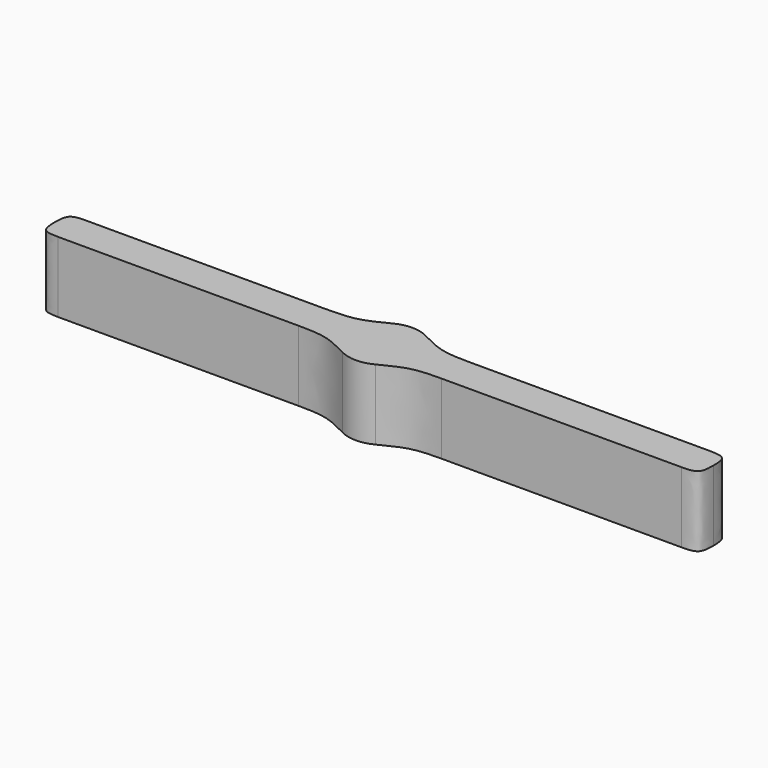
from build123d import *

# Parameters (mm, degrees)
F0_R        = 7.9375
F1_DEPTH    = 38.1
F2_T1_DEPTH = 85.725
F3_T1_DEPTH = 38.1


# Not quite as in the source:
# - a fillet or chamfer that OpenCascade refuses, or shapes differently, is made with other operations: its cross-section is extruded or revolved along the edge and cut away or added
# - a length typed as a fraction of an inch, garbled in the dataset ("3 / 203.2 mm" for 3/8 in), is restored


with BuildPart() as f1:
    # F0 (on Top) → F1 (new body)
    with BuildSketch(Plane.XY):
        with BuildLine():
            Line((16.4977839421, -9.525), (177.8, -9.525))
            Line((177.8, -9.525), (177.8, 9.525))
            Line((177.8, 9.525), (16.4977839421, 9.525))
            ThreePointArc((16.4977839421, 9.525), (0, 19.05), (-16.4977839421, 9.525))
            Line((-16.4977839421, 9.525), (-177.8, 9.525))
            Line((-177.8, 9.525), (-177.8, -9.525))
            Line((-177.8, -9.525), (-16.4977839421, -9.525))
            ThreePointArc((-16.4977839421, -9.525), (0, -19.05), (16.4977839421, -9.525))
        make_face()
        Circle(F0_R, mode=Mode.SUBTRACT)
        Circle(F0_R)
    extrude(amount=F1_DEPTH)

    # F2: fillet of radius 9.525 on 4 edges, made by hand

    # F2_s2 → F2_t1 (cut)
    with BuildSketch(Plane.XY.offset(-23.8125)):
        with BuildLine():
            add(Edge.make_bspline(
                [(-177.8, 0), (-177.8, -9.525), (-168.275, -9.525)],
                knots=[0, 0, 0, 1, 1, 1], degree=2, weights=[1, 1.8571428571, 1]))
            Line((-168.275, -9.525), (-177.8, -9.525))
            Line((-177.8, -9.525), (-177.8, 0))
        make_face()
        with BuildLine():
            add(Edge.make_bspline(
                [(-168.275, 9.525), (-177.8, 9.525), (-177.8, 0)],
                knots=[0, 0, 0, 1, 1, 1], degree=2, weights=[1, 1.8571428571, 1]))
            Line((-177.8, 0), (-177.8, 9.525))
            Line((-177.8, 9.525), (-168.275, 9.525))
        make_face()
        with BuildLine():
            add(Edge.make_bspline(
                [(177.8, 0), (177.8, 9.525), (168.275, 9.525)],
                knots=[0, 0, 0, 1, 1, 1], degree=2, weights=[1, 1.8571428571, 1]))
            Line((168.275, 9.525), (177.8, 9.525))
            Line((177.8, 9.525), (177.8, 0))
        make_face()
        with BuildLine():
            add(Edge.make_bspline(
                [(168.275, -9.525), (177.8, -9.525), (177.8, 0)],
                knots=[0, 0, 0, 1, 1, 1], degree=2, weights=[1, 1.8571428571, 1]))
            Line((177.8, 0), (177.8, -9.525))
            Line((177.8, -9.525), (168.275, -9.525))
        make_face()
    extrude(amount=F2_T1_DEPTH, mode=Mode.SUBTRACT)

    # F3: fillet of radius 64.0333905996 on 4 edges, made by hand

    # F3_s2 → F3_t1 (join)
    with BuildSketch(Plane.XY):
        with BuildLine():
            add(Edge.make_bspline(
                [(8.8566007427, 16.8660346046), (22.8364726227, 9.525), (38.6265836688, 9.525)],
                knots=[0, 0, 0, 1, 1, 1], degree=2, weights=[1, 1.8571428571, 1]))
            Line((38.6265836688, 9.525), (16.4977839421, 9.525))
            ThreePointArc((16.4977839421, 9.525), (13.1978749408, 13.737488746), (8.8566007427, 16.8660346046))
        make_face()
        with BuildLine():
            add(Edge.make_bspline(
                [(-38.6265836688, 9.525), (-22.8364726227, 9.525), (-8.8566007427, 16.8660346046)],
                knots=[0, 0, 0, 1, 1, 1], degree=2, weights=[1, 1.8571428571, 1]))
            ThreePointArc((-8.8566007427, 16.8660346046), (-13.1978749408, 13.737488746), (-16.4977839421, 9.525))
            Line((-16.4977839421, 9.525), (-38.6265836688, 9.525))
        make_face()
        with BuildLine():
            add(Edge.make_bspline(
                [(-8.8566007427, -16.8660346046), (-22.8364726227, -9.525), (-38.6265836688, -9.525)],
                knots=[0, 0, 0, 1, 1, 1], degree=2, weights=[1, 1.8571428571, 1]))
            Line((-38.6265836688, -9.525), (-16.4977839421, -9.525))
            ThreePointArc((-16.4977839421, -9.525), (-13.1978749408, -13.737488746), (-8.8566007427, -16.8660346046))
        make_face()
        with BuildLine():
            add(Edge.make_bspline(
                [(8.8566007427, -16.8660346046), (22.8364726227, -9.525), (38.6265836688, -9.525)],
                knots=[0, 0, 0, 1, 1, 1], degree=2, weights=[1, 1.8571428571, 1]))
            Line((38.6265836688, -9.525), (16.4977839421, -9.525))
            ThreePointArc((16.4977839421, -9.525), (13.1978749408, -13.737488746), (8.8566007427, -16.8660346046))
        make_face()
    extrude(amount=F3_T1_DEPTH)


solid = f1.part
